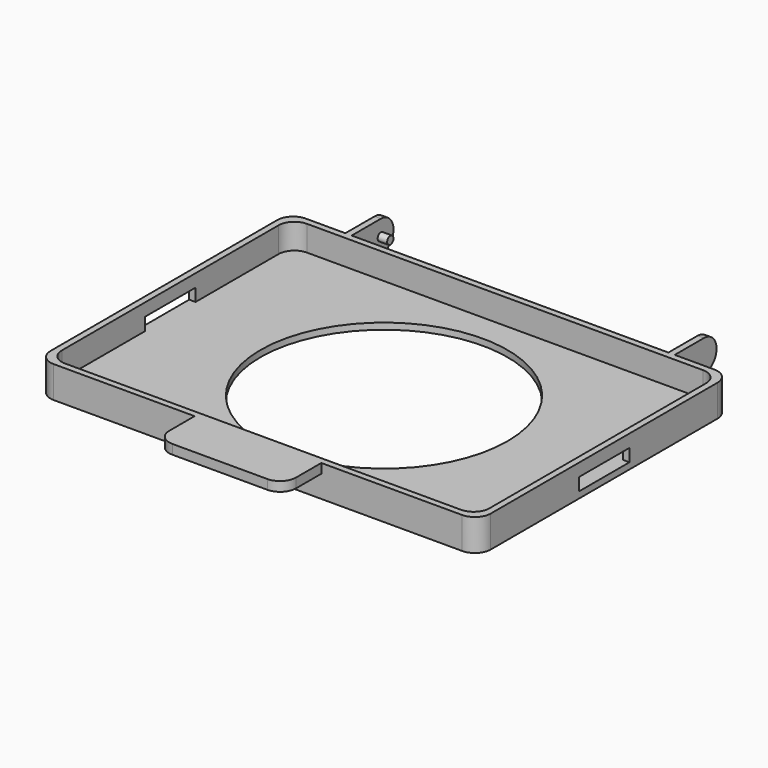
from build123d import *

# Parameters (mm, degrees)
F1_DEPTH  = 10
F0_R      = 39
F2_DEPTH  = 2
F4_DEPTH  = 3
F5_W      = 20
F5_H      = 4
F6_DEPTH  = 2
F7_W      = 20
F7_H      = 4
F8_DEPTH  = 2
F9_W      = 2
F9_H      = 10
F10_DEPTH = 11.5
F12_DEPTH = 2
F13_R     = 1.25
F14_DEPTH = 3
F16_R     = 1.25
F17_DEPTH = 2
F18_DEPTH = 5


# Not quite as in the source:
# - a feature names something its author has since deleted; it is built from what else it names


with BuildPart() as f1:
    # F0 (on Top) → F1 (new body)
    with BuildSketch(Plane.XY):
        with BuildLine():
            ThreePointArc((69.5, 44.75), (68.0355339059, 48.2855339059), (64.5, 49.75))
            Line((64.5, 49.75), (-64.5, 49.75))
            ThreePointArc((-64.5, 49.75), (-68.0355339059, 48.2855339059), (-69.5, 44.75))
            Line((-69.5, 44.75), (-69.5, -44.75))
            ThreePointArc((-69.5, -44.75), (-68.0355339059, -48.2855339059), (-64.5, -49.75))
            Line((-64.5, -49.75), (64.5, -49.75))
            ThreePointArc((64.5, -49.75), (68.0355339059, -48.2855339059), (69.5, -44.75))
            Line((69.5, -44.75), (69.5, 44.75))
        make_face()
        with BuildLine():
            Line((-62.5, 47.75), (62.5, 47.75))
            ThreePointArc((62.5, 47.75), (66.0355339059, 46.2855339059), (67.5, 42.75))
            Line((67.5, 42.75), (67.5, -42.75))
            ThreePointArc((67.5, -42.75), (66.0355339059, -46.2855339059), (62.5, -47.75))
            Line((62.5, -47.75), (-62.5, -47.75))
            ThreePointArc((-62.5, -47.75), (-66.0355339059, -46.2855339059), (-67.5, -42.75))
            Line((-67.5, -42.75), (-67.5, 42.75))
            ThreePointArc((-67.5, 42.75), (-66.0355339059, 46.2855339059), (-62.5, 47.75))
        make_face(mode=Mode.SUBTRACT)
    extrude(amount=F1_DEPTH)

    # F0 (on Top) → F2 (join)
    with BuildSketch(Plane.XY):
        with BuildLine():
            ThreePointArc((67.5, 42.75), (66.0355339059, 46.2855339059), (62.5, 47.75))
            Line((62.5, 47.75), (-62.5, 47.75))
            ThreePointArc((-62.5, 47.75), (-66.0355339059, 46.2855339059), (-67.5, 42.75))
            Line((-67.5, 42.75), (-67.5, -42.75))
            ThreePointArc((-67.5, -42.75), (-66.0355339059, -46.2855339059), (-62.5, -47.75))
            Line((-62.5, -47.75), (62.5, -47.75))
            ThreePointArc((62.5, -47.75), (66.0355339059, -46.2855339059), (67.5, -42.75))
            Line((67.5, -42.75), (67.5, 42.75))
        make_face()
        Circle(F0_R, mode=Mode.SUBTRACT)
    extrude(amount=F2_DEPTH)

    # F3 (on face) → F4 (join)
    with BuildSketch(Plane.XY.offset(10)):
        with BuildLine():
            Line((20, -49.75), (-20, -49.75))
            Line((-20, -49.75), (-20, -59.75))
            ThreePointArc((-20, -59.75), (-18.5355339059, -63.2855339059), (-15, -64.75))
            Line((-15, -64.75), (15, -64.75))
            ThreePointArc((15, -64.75), (18.5355339059, -63.2855339059), (20, -59.75))
            Line((20, -59.75), (20, -49.75))
        make_face()
    extrude(amount=-F4_DEPTH)

    # F5 (on face) → F6 (cut, through all)
    with BuildSketch(Plane.YZ.offset(-67.5)):
        with Locations((0, 4)):
            Rectangle(F5_W, F5_H)
    extrude(amount=-F6_DEPTH, mode=Mode.SUBTRACT)

    # F7 (on face) → F8 (cut, through all)
    with BuildSketch(Plane(origin=(67.5, 0, 0), x_dir=(0, -1, 0), z_dir=(-1, 0, 0))):
        with Locations((0, 4)):
            Rectangle(F7_W, F7_H)
    extrude(amount=-F8_DEPTH, mode=Mode.SUBTRACT)

    # F9 (on face) → F10 (join)
    with BuildSketch(Plane(origin=(0, 49.75, 0), x_dir=(-1, 0, 0), z_dir=(0, 1, 0))):
        with Locations((51, 5)):
            Rectangle(F9_W, F9_H)
    extrude(amount=F10_DEPTH)

    # F11 (on face) → F12 (join)
    with BuildSketch(Plane(origin=(-52, 0, 0), x_dir=(0, -1, 0), z_dir=(-1, 0, 0))):
        with BuildLine():
            Line((-61.25, 0), (-61.25, 10))
            ThreePointArc((-61.25, 10), (-66.25, 5), (-61.25, 0))
        make_face()
    extrude(amount=-F12_DEPTH)

    # F13 (on face) → F14 (join)
    with BuildSketch(Plane.YZ.offset(-50)):
        with Locations((61.25, 5)):
            Circle(F13_R)
    extrude(amount=F14_DEPTH)

    # F16 (on offset) → F17 (join)
    with BuildSketch(Plane.YZ.offset(52)):
        with BuildLine():
            Line((61.25, 10), (49.75, 10))
            Line((49.75, 10), (49.75, 0))
            Line((49.75, 0), (61.25, 0))
            ThreePointArc((61.25, 0), (66.25, 5), (61.25, 10))
        make_face()
        with Locations((61.25, 5)):
            Circle(F16_R, mode=Mode.SUBTRACT)
    extrude(amount=-F17_DEPTH)

    # F16 (on offset) → F18 (join)
    with BuildSketch(Plane.YZ.offset(52)):
        with Locations((61.25, 5)):
            Circle(F16_R)
    extrude(amount=-F18_DEPTH)


solid = f1.part
